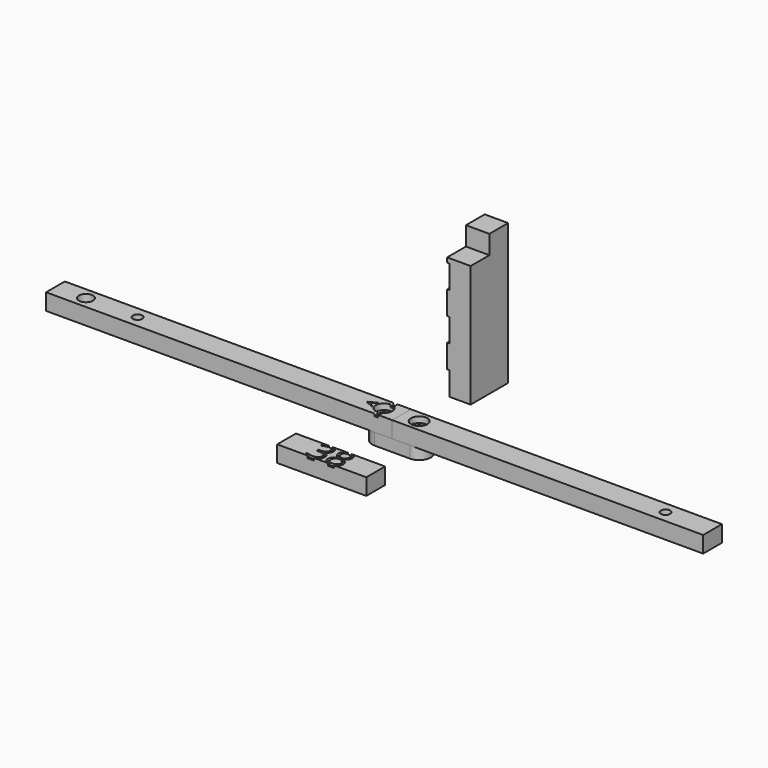
from build123d import *

# Parameters (mm, degrees)
F0_R          = 3
F0_R_2        = 2
F1_DEPTH      = 7
F2_DEPTH      = 7
F3_R          = 3.5
F4_DEPTH      = 2.5
F5_R          = 3.5
F5_R_2        = 2
F6_DEPTH      = 2.5
F7_R          = 1.5
F8_DEPTH      = 5
F9_W          = 10
F9_H          = 20
F10_DEPTH     = 60
F11_W         = 10
F11_H         = 8
F12_DEPTH     = 137.501
F13_W         = 38
F13_H         = 10
F14_DEPTH     = 7
F15_W         = 20
F15_H         = 10
F16_DEPTH     = 1
F18_DEPTH     = 1
F19_W         = 1.5
F19_H         = 10
F19_TEXT_SIZE = 6.8792319831
F20_DEPTH     = 1
F21_R         = 0.5
F22_R         = 0.8


# Not quite as in the source:
# - Text() gives the source's letters only with a copy of the font that has no kerning and outlines rounded to 1/6400 em; it was checked with that copy


with BuildPart() as f1:
    # F0 (on Top) → F1 (new body)
    with BuildSketch(Plane.XY):
        Polygon((0, 0), (0, 5), (-140, 5), (-147.5, 5), (-147.5, 0), (-147.5, -5), (-140, -5), (0, -5), align=None)
        with Locations((-134.5, 0)):
            Circle(F0_R, mode=Mode.SUBTRACT)
        with Locations((-112.5, 0)):
            Circle(F0_R_2, mode=Mode.SUBTRACT)
        with Locations((-7.5, 0)):
            Circle(F0_R_2, mode=Mode.SUBTRACT)
    extrude(amount=F1_DEPTH)

    # F3 (on face) → F4 (cut)
    with BuildSketch(Plane.XY.offset(7)):
        with Locations((-7.5, 0)):
            Circle(F3_R)
    extrude(amount=-F4_DEPTH, mode=Mode.SUBTRACT)

    # F19 (on face) → F20 (cut)
    with BuildSketch(Plane.XY.offset(7)):
        with Locations((-6.75, 0)):
            Rectangle(F19_W, F19_H)
        with Locations((-15.0507790968, -2.3359684274)):
            Text('<', F19_TEXT_SIZE, font='Open Sans', text_align=(TextAlign.LEFT, TextAlign.BOTTOM))
    extrude(amount=-F20_DEPTH, mode=Mode.SUBTRACT)

    # F21
    f21_edges = [f1.edges().sort_by_distance(p)[0] for p in [
        (-7.5, 4.25, 7),
        (-6, 4.081139, 7),
        (-7.5, -4.25, 7),
        (-6, -4.081139, 7),
    ]]
    fillet(f21_edges, radius=F21_R)

    # F22
    f22_edges = [f1.edges().sort_by_distance(p)[0] for p in [
        (-14.100585, 0.085736, 6.5),
    ]]
    fillet(f22_edges, radius=F22_R)


with BuildPart() as f2:
    # F0 (on Top) → F2 (new body)
    with BuildSketch(Plane.XY):
        Polygon((132.5, 0), (132.5, 5), (0, 5), (0, 0), (0, -5), (132.5, -5), align=None)
        with Locations((7.5, 0)):
            Circle(F0_R_2, mode=Mode.SUBTRACT)
        with Locations((112.5, 0)):
            Circle(F0_R_2, mode=Mode.SUBTRACT)
    extrude(amount=F2_DEPTH)

    # F5 (on face) → F6 (cut)
    with BuildSketch(Plane.XY.offset(7)):
        with Locations((7.5, 0)):
            Circle(F5_R)
        with Locations((7.5, 0)):
            Circle(F5_R_2, mode=Mode.SUBTRACT)
    extrude(amount=-F6_DEPTH, mode=Mode.SUBTRACT)


with BuildPart() as f8:
    # F7 (on Top) → F8 (new body)
    with BuildSketch(Plane.XY):
        with BuildLine():
            Line((-7.5, -5), (0, -5))
            Line((0, -5), (7.5, -5))
            ThreePointArc((7.5, -5), (12.5, 0), (7.5, 5))
            Line((7.5, 5), (0, 5))
            Line((0, 5), (-7.5, 5))
            ThreePointArc((-7.5, 5), (-12.5, 0), (-7.5, -5))
        make_face()
        with Locations((-7.5, 0)):
            Circle(F7_R, mode=Mode.SUBTRACT)
        with Locations((7.5, 0)):
            Circle(F7_R, mode=Mode.SUBTRACT)
    extrude(amount=-F8_DEPTH)


with BuildPart() as f10:
    # F9 (on Top) → F10 (new body)
    with BuildSketch(Plane.XY):
        with Locations((0, 40.5141524971)):
            Rectangle(F9_W, F9_H)
    extrude(amount=F10_DEPTH)

    # F11 (on face) → F12 (cut, through all)
    with BuildSketch(Plane(origin=(-5, 0, 0), x_dir=(0, -1, 0), z_dir=(-1, 0, 0))):
        with Locations((-35.5141524971, 56)):
            Rectangle(F11_W, F11_H)
    extrude(amount=-F12_DEPTH, mode=Mode.SUBTRACT)

    # F15 (on face) → F16 (cut)
    with BuildSketch(Plane(origin=(-5, 0, 0), x_dir=(0, -1, 0), z_dir=(-1, 0, 0))):
        with Locations((-40.5141524971, 45)):
            Rectangle(F15_W, F15_H)
        with Locations((-40.5141524971, 25)):
            Rectangle(F15_W, F15_H)
        with Locations((-40.5141524971, 5)):
            Rectangle(F15_W, F15_H)
    extrude(amount=-F16_DEPTH, mode=Mode.SUBTRACT)


with BuildPart() as f14:
    # F13 (on Top) → F14 (new body)
    with BuildSketch(Plane.XY):
        with Locations((0, -37.5424548984)):
            Rectangle(F13_W, F13_H)
    extrude(amount=F14_DEPTH)

    # F17 (on face) → F18 (cut)
    with BuildSketch(Plane.XY.offset(7)):
        with BuildLine():
            Line((4.6938740165, -32.5424548984), (3.1866145463, -32.5424548984))
            add(Edge.make_bspline(
                [(1.7994811469, -33.1262212164), (2.3594754098, -32.6760895881), (3.1866145463, -32.5424548984)],
                knots=[0, 0, 0, 0.7031208621, 0.7031208621, 0.7031208621], degree=2))
            add(Edge.make_bspline(
                [(1.0030401746, -34.8449712164), (1.0030401746, -33.7664121886), (1.7994811469, -33.1262212164)],
                knots=[0, 0, 0, 1, 1, 1], degree=2))
            add(Edge.make_bspline(
                [(1.4099412163, -36.2186691331), (1.0030401746, -35.6045198275), (1.0030401746, -34.8449712164)],
                knots=[0, 0, 0, 1, 1, 1], degree=2))
            add(Edge.make_bspline(
                [(2.7521721191, -37.3601621886), (1.816842258, -36.8328184386), (1.4099412163, -36.2186691331)],
                knots=[0, 0, 0, 1, 1, 1], degree=2))
            add(Edge.make_bspline(
                [(0.6775193413, -40.0120719108), (0.6775193413, -38.3106830219), (2.7521721191, -37.3601621886)],
                knots=[0, 0, 0, 1, 1, 1], degree=2))
            add(Edge.make_bspline(
                [(1.5325540635, -41.9836430914), (0.6775193413, -41.2881135775), (0.6775193413, -40.0120719108)],
                knots=[0, 0, 0, 1, 1, 1], degree=2))
            add(Edge.make_bspline(
                [(2.7110553463, -42.5424548984), (2.0085022562, -42.3708039943), (1.5325540635, -41.9836430914)],
                knots=[0.4433580528, 0.4433580528, 0.4433580528, 1, 1, 1], degree=2))
            Line((2.7110553463, -42.5424548984), (5.1460444464, -42.5424548984))
            add(Edge.make_bspline(
                [(6.3329012858, -41.9424104525), (5.842486748, -42.3617951769), (5.1460444464, -42.5424548984)],
                knots=[0, 0, 0, 0.5692267481, 0.5692267481, 0.5692267481], degree=2))
            add(Edge.make_bspline(
                [(7.1944464246, -39.9730094108), (7.1944464246, -41.2056482997), (6.3329012858, -41.9424104525)],
                knots=[0, 0, 0, 1, 1, 1], degree=2))
            add(Edge.make_bspline(
                [(6.6855488552, -38.5038253831), (7.1944464246, -39.1375059386), (7.1944464246, -39.9730094108)],
                knots=[0, 0, 0, 1, 1, 1], degree=2))
            add(Edge.make_bspline(
                [(4.9700540635, -37.2928878831), (6.1766512858, -37.8701448275), (6.6855488552, -38.5038253831)],
                knots=[0, 0, 0, 1, 1, 1], degree=2))
            add(Edge.make_bspline(
                [(6.4218769802, -36.1947976053), (5.9683179524, -36.7980962164), (4.9700540635, -37.2928878831)],
                knots=[0, 0, 0, 1, 1, 1], degree=2))
            add(Edge.make_bspline(
                [(6.875436008, -34.8579920497), (6.875436008, -35.5914989942), (6.4218769802, -36.1947976053)],
                knots=[0, 0, 0, 1, 1, 1], degree=2))
            add(Edge.make_bspline(
                [(6.0822502441, -33.1164555914), (6.875436008, -33.7468809386), (6.875436008, -34.8579920497)],
                knots=[0, 0, 0, 1, 1, 1], degree=2))
            add(Edge.make_bspline(
                [(4.6938740165, -32.5424548984), (5.5263616349, -32.6746344122), (6.0822502441, -33.1164555914)],
                knots=[0.2991697096, 0.2991697096, 0.2991697096, 1, 1, 1], degree=2))
        make_face()
        with BuildLine():
            add(Edge.make_bspline(
                [(1.7908005913, -40.0402837164), (1.7908005913, -40.8540857997), (2.3561217719, -41.3087298969)],
                knots=[0, 0, 0, 1, 1, 1], degree=2))
            add(Edge.make_bspline(
                [(2.2443596191, -38.7816031608), (1.7908005913, -39.3067767719), (1.7908005913, -40.0402837164)],
                knots=[0, 0, 0, 1, 1, 1], degree=2))
            add(Edge.make_bspline(
                [(3.7092033691, -37.8224017719), (2.6979186469, -38.2564295497), (2.2443596191, -38.7816031608)],
                knots=[0, 0, 0, 1, 1, 1], degree=2))
            add(Edge.make_bspline(
                [(5.5538214246, -38.8163253831), (5.0243075358, -38.3041726053), (3.7092033691, -37.8224017719)],
                knots=[0, 0, 0, 1, 1, 1], degree=2))
            add(Edge.make_bspline(
                [(6.0833353135, -39.9860302442), (6.0833353135, -39.3284781608), (5.5538214246, -38.8163253831)],
                knots=[0, 0, 0, 1, 1, 1], degree=2))
            add(Edge.make_bspline(
                [(5.5201842719, -41.2881135775), (6.0833353135, -40.8128531608), (6.0833353135, -39.9860302442)],
                knots=[0, 0, 0, 1, 1, 1], degree=2))
            add(Edge.make_bspline(
                [(3.945748508, -41.7633739942), (4.9570332302, -41.7633739942), (5.5201842719, -41.2881135775)],
                knots=[0, 0, 0, 1, 1, 1], degree=2))
            add(Edge.make_bspline(
                [(2.3561217719, -41.3087298969), (2.9214429524, -41.7633739942), (3.945748508, -41.7633739942)],
                knots=[0, 0, 0, 1, 1, 1], degree=2))
        make_face(mode=Mode.SUBTRACT)
        with BuildLine():
            add(Edge.make_bspline(
                [(3.9197068413, -33.3996587164), (3.0711825358, -33.3996587164), (2.5894117024, -33.8065597581)],
                knots=[0, 0, 0, 1, 1, 1], degree=2))
            add(Edge.make_bspline(
                [(5.2727884385, -33.8033045497), (4.7812519802, -33.3996587164), (3.9197068413, -33.3996587164)],
                knots=[0, 0, 0, 1, 1, 1], degree=2))
            add(Edge.make_bspline(
                [(5.7643248969, -34.8927142719), (5.7643248969, -34.2069503831), (5.2727884385, -33.8033045497)],
                knots=[0, 0, 0, 1, 1, 1], degree=2))
            add(Edge.make_bspline(
                [(5.3606790635, -35.9842941331), (5.7643248969, -35.5155441331), (5.7643248969, -34.8927142719)],
                knots=[0, 0, 0, 1, 1, 1], degree=2))
            add(Edge.make_bspline(
                [(3.9869811469, -36.8588601053), (4.9570332302, -36.4530441331), (5.3606790635, -35.9842941331)],
                knots=[0, 0, 0, 1, 1, 1], degree=2))
            add(Edge.make_bspline(
                [(2.5080314941, -35.9636778136), (2.9084221191, -36.4118114942), (3.9869811469, -36.8588601053)],
                knots=[0, 0, 0, 1, 1, 1], degree=2))
            add(Edge.make_bspline(
                [(2.1076408691, -34.8927142719), (2.1076408691, -35.5155441331), (2.5080314941, -35.9636778136)],
                knots=[0, 0, 0, 1, 1, 1], degree=2))
            add(Edge.make_bspline(
                [(2.5894117024, -33.8065597581), (2.1076408691, -34.2134607997), (2.1076408691, -34.8927142719)],
                knots=[0, 0, 0, 1, 1, 1], degree=2))
        make_face(mode=Mode.SUBTRACT)
        with BuildLine():
            add(Edge.make_bspline(
                [(-1.1453973254, -34.9599885775), (-1.1453973254, -35.9105094108), (-1.6781664226, -36.5138080219)],
                knots=[0, 0, 0, 1, 1, 1], degree=2))
            add(Edge.make_bspline(
                [(-1.9461785754, -33.1468375358), (-1.1453973254, -33.8076448275), (-1.1453973254, -34.9599885775)],
                knots=[0, 0, 0, 1, 1, 1], degree=2))
            add(Edge.make_bspline(
                [(-3.4015466925, -32.5424548984), (-2.5129624773, -32.6791256168), (-1.9461785754, -33.1468375358)],
                knots=[0.2922113225, 0.2922113225, 0.2922113225, 1, 1, 1], degree=2))
            Line((-3.4015466925, -32.5424548984), (-4.9731217949, -32.5424548984))
            add(Edge.make_bspline(
                [(-5.8697896865, -32.7605528136), (-5.434425044, -32.6104884341), (-4.9731217949, -32.5424548984)],
                knots=[0, 0, 0, 0.5466376764, 0.5466376764, 0.5466376764], degree=2))
            add(Edge.make_bspline(
                [(-7.2760396865, -33.5168462164), (-6.6662306587, -33.0350753831), (-5.8697896865, -32.7605528136)],
                knots=[0, 0, 0, 1, 1, 1], degree=2))
            Line((-7.2760396865, -33.5168462164), (-6.7074632976, -34.2763948275))
            add(Edge.make_bspline(
                [(-5.3912740615, -33.6242680914), (-5.9674459365, -33.8011344108), (-6.7074632976, -34.2763948275)],
                knots=[0, 0, 0, 1, 1, 1], degree=2))
            add(Edge.make_bspline(
                [(-4.1640605198, -33.4474017719), (-4.8151021865, -33.4474017719), (-5.3912740615, -33.6242680914)],
                knots=[0, 0, 0, 1, 1, 1], degree=2))
            add(Edge.make_bspline(
                [(-2.8109789226, -33.8618982997), (-3.3090257976, -33.4474017719), (-4.1640605198, -33.4474017719)],
                knots=[0, 0, 0, 1, 1, 1], degree=2))
            add(Edge.make_bspline(
                [(-2.3129320476, -35.0012212164), (-2.3129320476, -34.2763948275), (-2.8109789226, -33.8618982997)],
                knots=[0, 0, 0, 1, 1, 1], degree=2))
            add(Edge.make_bspline(
                [(-2.9911004504, -36.4226621886), (-2.3129320476, -35.9105094108), (-2.3129320476, -35.0012212164)],
                knots=[0, 0, 0, 1, 1, 1], degree=2))
            add(Edge.make_bspline(
                [(-4.8281230198, -36.9348149664), (-3.6692688531, -36.9348149664), (-2.9911004504, -36.4226621886)],
                knots=[0, 0, 0, 1, 1, 1], degree=2))
            Line((-4.8281230198, -36.9348149664), (-5.8177063531, -36.9348149664))
            Line((-5.8177063531, -36.9348149664), (-5.8177063531, -37.9026969108))
            Line((-5.8177063531, -37.9026969108), (-4.8411438531, -37.9026969108))
            add(Edge.make_bspline(
                [(-2.0069424642, -39.7082524664), (-2.0069424642, -37.9026969108), (-4.8411438531, -37.9026969108)],
                knots=[0, 0, 0, 1, 1, 1], degree=2))
            add(Edge.make_bspline(
                [(-4.5763869087, -41.7221413553), (-2.0069424642, -41.7221413553), (-2.0069424642, -39.7082524664)],
                knots=[0, 0, 0, 1, 1, 1], degree=2))
            add(Edge.make_bspline(
                [(-5.956595242, -41.5561257303), (-5.2274285754, -41.7221413553), (-4.5763869087, -41.7221413553)],
                knots=[0, 0, 0, 1, 1, 1], degree=2))
            add(Edge.make_bspline(
                [(-7.3302931587, -41.0710996886), (-6.6857619087, -41.3901101053), (-5.956595242, -41.5561257303)],
                knots=[0, 0, 0, 1, 1, 1], degree=2))
            Line((-7.3302931587, -41.0710996886), (-7.3302931587, -42.1431482997))
            add(Edge.make_bspline(
                [(-6.149994361, -42.5424548984), (-6.7565968671, -42.4198961587), (-7.3302931587, -42.1431482997)],
                knots=[0.0691575663, 0.0691575663, 0.0691575663, 1, 1, 1], degree=2))
            Line((-6.149994361, -42.5424548984), (-3.2342283647, -42.5424548984))
            add(Edge.make_bspline(
                [(-1.8246507976, -41.9152837164), (-2.3918293667, -42.3560052535), (-3.2342283647, -42.5424548984)],
                knots=[0, 0, 0, 0.5769445577, 0.5769445577, 0.5769445577], degree=2))
            add(Edge.make_bspline(
                [(-0.8415778809, -39.7342941331), (-0.8415778809, -41.1513948275), (-1.8246507976, -41.9152837164)],
                knots=[0, 0, 0, 1, 1, 1], degree=2))
            add(Edge.make_bspline(
                [(-1.4177497559, -38.1338167025), (-0.8415778809, -38.7447107997), (-0.8415778809, -39.7342941331)],
                knots=[0, 0, 0, 1, 1, 1], degree=2))
            add(Edge.make_bspline(
                [(-3.1874980198, -37.3753531608), (-1.9939216309, -37.5229226053), (-1.4177497559, -38.1338167025)],
                knots=[0, 0, 0, 1, 1, 1], degree=2))
            Line((-3.1874980198, -37.3753531608), (-3.1874980198, -37.3210996886))
            add(Edge.make_bspline(
                [(-1.6781664226, -36.5138080219), (-2.2109355198, -37.1171066331), (-3.1874980198, -37.3210996886)],
                knots=[0, 0, 0, 1, 1, 1], degree=2))
        make_face()
    extrude(amount=-F18_DEPTH, mode=Mode.SUBTRACT)


solid = Compound([f1.part, f2.part, f8.part, f10.part, f14.part])
